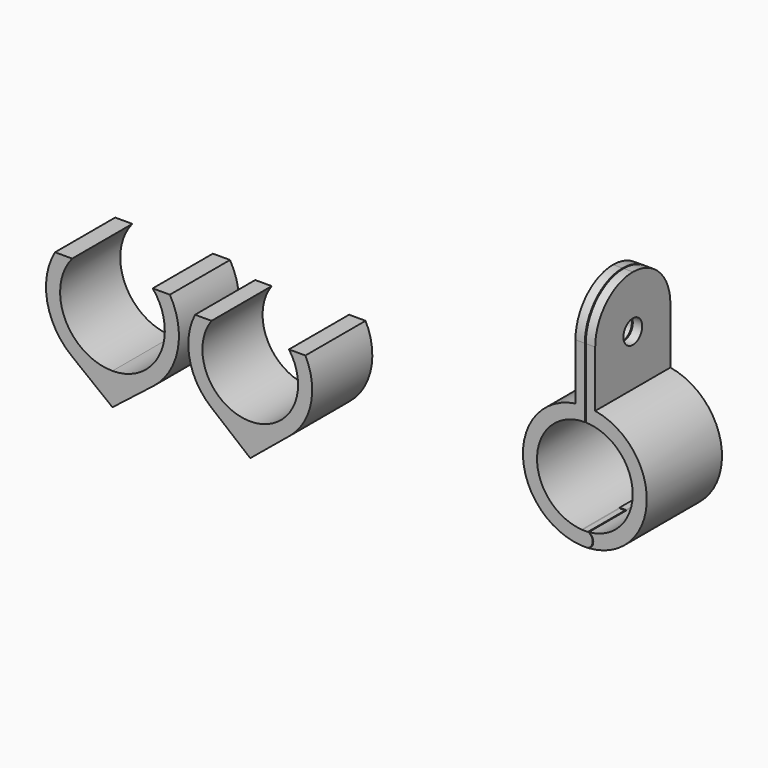
from build123d import *

# Parameters (mm, degrees)
F5_DEPTH  = 5
F0_R      = 0.45
F6_DEPTH  = 3.5
F7_DEPTH  = 5
F8_DEPTH  = 3.3
F9_DEPTH  = 5.001
F10_DEPTH = 8.001
F11_DEPTH = 0.05
F12_R     = 1.25
F13_DEPTH = 62.4297639076
F14_R     = 4.99999


# Not quite as in the source:
# - a fillet or chamfer is up to 0.001 mm smaller than in the source, because OpenCascade refuses the exact size
# - a feature names something its author has since deleted; it is built from what else it names


with BuildPart() as f3:
    # F3: sweep along a path in F2
    with BuildLine(Plane.XY) as f3_path:
        Line((0, 0), (0, 8))
    # F0 (on Front) → F3 (sweep)
    with BuildSketch(Plane.XZ):
        with BuildLine():
            Line((-4.2852259595, 12.5322833964), (-6.1092684933, 12.5322833964))
            ThreePointArc((-6.1092684933, 12.5322833964), (-6.9428544736, 7.6391569536), (-4.3543082114, 3.4039497307))
            Line((-4.3543082114, 3.4039497307), (0, 3.4039497307))
            ThreePointArc((0, 3.4039497307), (-5.042063988, 6.6069916109), (-4.2852259595, 12.5322833964))
        make_face()
        with BuildLine():
            Line((0, 3.4039497307), (-4.3543082114, 3.4039497307))
            ThreePointArc((-4.3543082114, 3.4039497307), (-2.3027157879, 2.2894602214), (0, 1.9039497307))
            Line((0, 1.9039497307), (0, 3.4039497307))
        make_face()
        with BuildLine():
            ThreePointArc((0, 1.9039497307), (-2.3027157879, 2.2894602214), (-4.3543082114, 3.4039497307))
            Line((-4.3543082114, 3.4039497307), (0, 0))
            Line((0, 0), (0, 1.9039497307))
        make_face()
        with BuildLine():
            ThreePointArc((4.3543082114, 3.4039497307), (2.3027157879, 2.2894602214), (0, 1.9039497307))
            Line((0, 1.9039497307), (0, 0))
            Line((0, 0), (4.3543082114, 3.4039497307))
        make_face()
        with BuildLine():
            Line((0, 3.4039497307), (0, 1.9039497307))
            ThreePointArc((0, 1.9039497307), (2.3027157879, 2.2894602214), (4.3543082114, 3.4039497307))
            Line((4.3543082114, 3.4039497307), (0, 3.4039497307))
        make_face()
        with BuildLine():
            ThreePointArc((4.2852259595, 12.5322833964), (5.042063988, 6.6069916109), (0, 3.4039497307))
            Line((0, 3.4039497307), (4.3543082114, 3.4039497307))
            ThreePointArc((4.3543082114, 3.4039497307), (6.9428544736, 7.6391569536), (6.1092684933, 12.5322833964))
            Line((6.1092684933, 12.5322833964), (4.2852259595, 12.5322833964))
        make_face()
    sweep(path=f3_path.line)

    # F0 (on Front) → F9 (cut, through all)
    with BuildSketch(Plane.XZ):
        with BuildLine():
            ThreePointArc((54.5868154242, 8.1161158316), (55.0876267464, 7.3630999101), (54.581783754, 6.6134547771))
            ThreePointArc((54.581783754, 6.6134547771), (54.6381547588, 6.6164632985), (54.6944979239, 6.6199545901))
            ThreePointArc((54.6944979239, 6.6199545901), (55.1524674782, 7.3759380646), (54.6800855939, 8.1230006335))
            ThreePointArc((54.6800855939, 8.1230006335), (54.6334663221, 8.1193440091), (54.5868154242, 8.1161158316))
        make_face()
    extrude(amount=F9_DEPTH, mode=Mode.SUBTRACT)

    # F0 (on Front) → F10 (cut, through all)
    with BuildSketch(Plane.XZ):
        with BuildLine():
            ThreePointArc((53.9199314878, 8.116823601), (53.3614179699, 7.3872965022), (53.862876759, 6.6174353327))
            ThreePointArc((53.862876759, 6.6174353327), (53.9147482987, 6.6145187306), (53.9666412198, 6.6120111547))
            ThreePointArc((53.9666412198, 6.6120111547), (53.4175421646, 7.3754821716), (54.0022997363, 8.1119985313))
            ThreePointArc((54.0022997363, 8.1119985313), (53.961105835, 8.1142441636), (53.9199314878, 8.116823601))
        make_face()
    extrude(amount=-F10_DEPTH, mode=Mode.SUBTRACT)


with BuildPart() as f4:
    # F4: sweep along a path in F2
    with BuildLine(Plane.XY) as f4_path:
        Line((14.6589075401, 0), (14.6589075401, 8))
    # F0 (on Front) → F4 (sweep)
    with BuildSketch(Plane.XZ):
        with BuildLine():
            Line((10.542163481, 11.5254557146), (8.7879977598, 11.5254557146))
            ThreePointArc((8.7879977598, 11.5254557146), (8.2076139721, 7.1870854906), (10.4732176329, 3.442043222))
            Line((10.4732176329, 3.442043222), (14.6589075401, 3.442043222))
            ThreePointArc((14.6589075401, 3.442043222), (10.1232394754, 6.2221048665), (10.542163481, 11.5254557146))
        make_face()
        with BuildLine():
            Line((14.6589075401, 3.442043222), (10.4732176329, 3.442043222))
            ThreePointArc((10.4732176329, 3.442043222), (12.4357341326, 2.3283668926), (14.6589075401, 1.942043222))
            Line((14.6589075401, 1.942043222), (14.6589075401, 3.442043222))
        make_face()
        with BuildLine():
            ThreePointArc((14.6589075401, 1.942043222), (12.4357341326, 2.3283668926), (10.4732176329, 3.442043222))
            Line((10.4732176329, 3.442043222), (14.6589075401, 0))
            Line((14.6589075401, 0), (14.6589075401, 1.942043222))
        make_face()
        with BuildLine():
            ThreePointArc((18.8445974474, 3.442043222), (16.8820809477, 2.3283668926), (14.6589075401, 1.942043222))
            Line((14.6589075401, 1.942043222), (14.6589075401, 0))
            Line((14.6589075401, 0), (18.8445974474, 3.442043222))
        make_face()
        with BuildLine():
            Line((14.6589075401, 3.442043222), (14.6589075401, 1.942043222))
            ThreePointArc((14.6589075401, 1.942043222), (16.8820809477, 2.3283668926), (18.8445974474, 3.442043222))
            Line((18.8445974474, 3.442043222), (14.6589075401, 3.442043222))
        make_face()
        with BuildLine():
            ThreePointArc((18.7756515993, 11.5254557146), (19.1945756049, 6.2221048665), (14.6589075401, 3.442043222))
            Line((14.6589075401, 3.442043222), (18.8445974474, 3.442043222))
            ThreePointArc((18.8445974474, 3.442043222), (21.1102011082, 7.1870854906), (20.5298173205, 11.5254557146))
            Line((20.5298173205, 11.5254557146), (18.7756515993, 11.5254557146))
        make_face()
    sweep(path=f4_path.line)


with BuildPart() as f5:
    # F0 (on Front) → F5 (new body)
    with BuildSketch(Plane.XZ):
        with BuildLine():
            Line((53.2587639076, 18.1863348766), (53.2587639076, 19.7092189305))
            ThreePointArc((53.2587639076, 19.7092189305), (47.6757687932, 12.8917648009), (53.862876759, 6.6174353327))
            ThreePointArc((53.862876759, 6.6174353327), (53.3614179699, 7.3872965022), (53.9199314878, 8.116823601))
            ThreePointArc((53.9199314878, 8.116823601), (49.1797007662, 12.8620403018), (53.2587639076, 18.1863348766))
        make_face()
        with BuildLine():
            Line((53.2587639076, 30.67503149), (53.2587639076, 19.7092189305))
            Line((53.2587639076, 19.7092189305), (53.2587639076, 18.1863348766))
            ThreePointArc((53.2587639076, 18.1863348766), (53.7563098464, 18.2606730117), (54.2587639076, 18.2855333378))
            Line((54.2587639076, 18.2855333378), (54.2587639076, 30.67503149))
            Line((54.2587639076, 30.67503149), (53.2587639076, 30.67503149))
        make_face()
    extrude(amount=-F5_DEPTH)



with BuildPart() as f5b:
    # F0 (on Front) → F5, piece 2 (new body)
    with BuildSketch(Plane.XZ):
        with BuildLine():
            ThreePointArc((54.0022997363, 8.1119985313), (53.4175421646, 7.3754821716), (53.9666412198, 6.6120111547))
            ThreePointArc((53.9666412198, 6.6120111547), (54.1126666567, 6.6071529911), (54.2587639076, 6.6055333378))
            Line((54.2587639076, 6.6055333378), (54.2587639076, 6.8555333378))
            ThreePointArc((54.2587639076, 6.8555333378), (53.7587639076, 7.3555333378), (54.2587639076, 7.8555333378))
            Line((54.2587639076, 7.8555333378), (54.2587639076, 8.1055333378))
            ThreePointArc((54.2587639076, 8.1055333378), (54.1304910833, 8.1071498929), (54.0022997363, 8.1119985313))
        make_face()
        with BuildLine():
            Line((54.2587639076, 6.8555333378), (54.2587639076, 6.6055333378))
            ThreePointArc((54.2587639076, 6.6055333378), (54.420322388, 6.6075139953), (54.581783754, 6.6134547771))
            ThreePointArc((54.581783754, 6.6134547771), (55.0876267464, 7.3630999101), (54.5868154242, 8.1161158316))
            ThreePointArc((54.5868154242, 8.1161158316), (54.4228749879, 8.1081796492), (54.2587639076, 8.1055333378))
            Line((54.2587639076, 8.1055333378), (54.2587639076, 7.8555333378))
            ThreePointArc((54.2587639076, 7.8555333378), (54.6123172982, 7.7090867284), (54.7587639076, 7.3555333378))
            ThreePointArc((54.7587639076, 7.3555333378), (54.6123172982, 7.0019799472), (54.2587639076, 6.8555333378))
        make_face()
        with BuildLine():
            ThreePointArc((54.5868154242, 8.1161158316), (55.0876267464, 7.3630999101), (54.581783754, 6.6134547771))
            ThreePointArc((54.581783754, 6.6134547771), (54.6381547588, 6.6164632985), (54.6944979239, 6.6199545901))
            ThreePointArc((54.6944979239, 6.6199545901), (55.1524674782, 7.3759380646), (54.6800855939, 8.1230006335))
            ThreePointArc((54.6800855939, 8.1230006335), (54.6334663221, 8.1193440091), (54.5868154242, 8.1161158316))
        make_face()
        with BuildLine():
            ThreePointArc((54.2587639076, 7.8555333378), (53.7587639076, 7.3555333378), (54.2587639076, 6.8555333378))
            ThreePointArc((54.2587639076, 6.8555333378), (54.6123172982, 7.0019799472), (54.7587639076, 7.3555333378))
            ThreePointArc((54.7587639076, 7.3555333378), (54.6123172982, 7.7090867284), (54.2587639076, 7.8555333378))
        make_face()
        with Locations((54.2587639076, 7.3555333378)):
            Circle(F0_R, mode=Mode.SUBTRACT)
        with BuildLine():
            ThreePointArc((54.6800855939, 8.1230006335), (55.1524674782, 7.3759380646), (54.6944979239, 6.6199545901))
            ThreePointArc((54.6944979239, 6.6199545901), (60.8402732623, 12.8611165114), (55.3587639076, 19.6930790283))
            Line((55.3587639076, 19.6930790283), (55.3587639076, 18.1652516397))
            ThreePointArc((55.3587639076, 18.1652516397), (59.3371796287, 12.8523223769), (54.6800855939, 8.1230006335))
        make_face()
        with BuildLine():
            Line((55.3587639076, 18.1652516397), (55.3587639076, 19.6930790283))
            Line((55.3587639076, 19.6930790283), (55.3587639076, 30.67503149))
            Line((55.3587639076, 30.67503149), (54.3587639076, 30.67503149))
            Line((54.3587639076, 30.67503149), (54.3587639076, 18.2845509247))
            ThreePointArc((54.3587639076, 18.2845509247), (54.8617216838, 18.24969419), (55.3587639076, 18.1652516397))
        make_face()
        with Locations((54.2587639076, 7.3555333378)):
            Circle(F0_R)
    extrude(amount=-F5_DEPTH)

    # F0 (on Front) → F6 (cut)
    with BuildSketch(Plane.XZ):
        with BuildLine():
            ThreePointArc((54.2587639076, 7.8555333378), (53.7587639076, 7.3555333378), (54.2587639076, 6.8555333378))
            ThreePointArc((54.2587639076, 6.8555333378), (54.6123172982, 7.0019799472), (54.7587639076, 7.3555333378))
            ThreePointArc((54.7587639076, 7.3555333378), (54.6123172982, 7.7090867284), (54.2587639076, 7.8555333378))
        make_face()
        with Locations((54.2587639076, 7.3555333378)):
            Circle(F0_R, mode=Mode.SUBTRACT)
        with Locations((54.2587639076, 7.3555333378)):
            Circle(F0_R)
    extrude(amount=-F6_DEPTH, mode=Mode.SUBTRACT)


with BuildPart() as f5_1:
    add(f5.part)

    add(f5b.part)  # F7 merges F5b
    # F0 (on Front) → F7 (join)
    with BuildSketch(Plane.XZ):
        with BuildLine():
            Line((53.2587639076, 18.1863348766), (53.2587639076, 19.7092189305))
            ThreePointArc((53.2587639076, 19.7092189305), (47.6757687932, 12.8917648009), (53.862876759, 6.6174353327))
            ThreePointArc((53.862876759, 6.6174353327), (53.3614179699, 7.3872965022), (53.9199314878, 8.116823601))
            ThreePointArc((53.9199314878, 8.116823601), (49.1797007662, 12.8620403018), (53.2587639076, 18.1863348766))
        make_face()
        with BuildLine():
            Line((53.2587639076, 30.67503149), (53.2587639076, 19.7092189305))
            Line((53.2587639076, 19.7092189305), (53.2587639076, 18.1863348766))
            ThreePointArc((53.2587639076, 18.1863348766), (53.7563098464, 18.2606730117), (54.2587639076, 18.2855333378))
            Line((54.2587639076, 18.2855333378), (54.2587639076, 30.67503149))
            Line((54.2587639076, 30.67503149), (53.2587639076, 30.67503149))
        make_face()
        with BuildLine():
            ThreePointArc((53.9199314878, 8.116823601), (53.3614179699, 7.3872965022), (53.862876759, 6.6174353327))
            ThreePointArc((53.862876759, 6.6174353327), (53.9147482987, 6.6145187306), (53.9666412198, 6.6120111547))
            ThreePointArc((53.9666412198, 6.6120111547), (53.4175421646, 7.3754821716), (54.0022997363, 8.1119985313))
            ThreePointArc((54.0022997363, 8.1119985313), (53.961105835, 8.1142441636), (53.9199314878, 8.116823601))
        make_face()
        with BuildLine():
            ThreePointArc((54.0022997363, 8.1119985313), (53.4175421646, 7.3754821716), (53.9666412198, 6.6120111547))
            ThreePointArc((53.9666412198, 6.6120111547), (54.1126666567, 6.6071529911), (54.2587639076, 6.6055333378))
            Line((54.2587639076, 6.6055333378), (54.2587639076, 6.8555333378))
            ThreePointArc((54.2587639076, 6.8555333378), (53.7587639076, 7.3555333378), (54.2587639076, 7.8555333378))
            Line((54.2587639076, 7.8555333378), (54.2587639076, 8.1055333378))
            ThreePointArc((54.2587639076, 8.1055333378), (54.1304910833, 8.1071498929), (54.0022997363, 8.1119985313))
        make_face()
        with BuildLine():
            Line((54.2587639076, 6.8555333378), (54.2587639076, 6.6055333378))
            ThreePointArc((54.2587639076, 6.6055333378), (54.420322388, 6.6075139953), (54.581783754, 6.6134547771))
            ThreePointArc((54.581783754, 6.6134547771), (55.0876267464, 7.3630999101), (54.5868154242, 8.1161158316))
            ThreePointArc((54.5868154242, 8.1161158316), (54.4228749879, 8.1081796492), (54.2587639076, 8.1055333378))
            Line((54.2587639076, 8.1055333378), (54.2587639076, 7.8555333378))
            ThreePointArc((54.2587639076, 7.8555333378), (54.6123172982, 7.7090867284), (54.7587639076, 7.3555333378))
            ThreePointArc((54.7587639076, 7.3555333378), (54.6123172982, 7.0019799472), (54.2587639076, 6.8555333378))
        make_face()
        with BuildLine():
            ThreePointArc((54.2587639076, 7.8555333378), (53.7587639076, 7.3555333378), (54.2587639076, 6.8555333378))
            ThreePointArc((54.2587639076, 6.8555333378), (54.6123172982, 7.0019799472), (54.7587639076, 7.3555333378))
            ThreePointArc((54.7587639076, 7.3555333378), (54.6123172982, 7.7090867284), (54.2587639076, 7.8555333378))
        make_face()
        with Locations((54.2587639076, 7.3555333378)):
            Circle(F0_R, mode=Mode.SUBTRACT)
        with BuildLine():
            ThreePointArc((54.6800855939, 8.1230006335), (55.1524674782, 7.3759380646), (54.6944979239, 6.6199545901))
            ThreePointArc((54.6944979239, 6.6199545901), (60.8402732623, 12.8611165114), (55.3587639076, 19.6930790283))
            Line((55.3587639076, 19.6930790283), (55.3587639076, 18.1652516397))
            ThreePointArc((55.3587639076, 18.1652516397), (59.3371796287, 12.8523223769), (54.6800855939, 8.1230006335))
        make_face()
        with BuildLine():
            Line((55.3587639076, 18.1652516397), (55.3587639076, 19.6930790283))
            Line((55.3587639076, 19.6930790283), (55.3587639076, 30.67503149))
            Line((55.3587639076, 30.67503149), (54.3587639076, 30.67503149))
            Line((54.3587639076, 30.67503149), (54.3587639076, 18.2845509247))
            ThreePointArc((54.3587639076, 18.2845509247), (54.8617216838, 18.24969419), (55.3587639076, 18.1652516397))
        make_face()
        with Locations((54.2587639076, 7.3555333378)):
            Circle(F0_R)
    extrude(amount=F7_DEPTH)

    # F0 (on Front) → F8 (join)
    with BuildSketch(Plane.XZ):
        with Locations((54.2587639076, 7.3555333378)):
            Circle(F0_R)
    extrude(amount=-F8_DEPTH)

    # F0 (on Front) → F11 (cut, symmetric)
    with BuildSketch(Plane.XZ):
        with BuildLine():
            Line((54.2587639076, 6.8555333378), (54.2587639076, 6.6055333378))
            ThreePointArc((54.2587639076, 6.6055333378), (54.420322388, 6.6075139953), (54.581783754, 6.6134547771))
            ThreePointArc((54.581783754, 6.6134547771), (55.0876267464, 7.3630999101), (54.5868154242, 8.1161158316))
            ThreePointArc((54.5868154242, 8.1161158316), (54.4228749879, 8.1081796492), (54.2587639076, 8.1055333378))
            Line((54.2587639076, 8.1055333378), (54.2587639076, 7.8555333378))
            ThreePointArc((54.2587639076, 7.8555333378), (54.6123172982, 7.7090867284), (54.7587639076, 7.3555333378))
            ThreePointArc((54.7587639076, 7.3555333378), (54.6123172982, 7.0019799472), (54.2587639076, 6.8555333378))
        make_face()
        with BuildLine():
            ThreePointArc((54.0022997363, 8.1119985313), (53.4175421646, 7.3754821716), (53.9666412198, 6.6120111547))
            ThreePointArc((53.9666412198, 6.6120111547), (54.1126666567, 6.6071529911), (54.2587639076, 6.6055333378))
            Line((54.2587639076, 6.6055333378), (54.2587639076, 6.8555333378))
            ThreePointArc((54.2587639076, 6.8555333378), (53.7587639076, 7.3555333378), (54.2587639076, 7.8555333378))
            Line((54.2587639076, 7.8555333378), (54.2587639076, 8.1055333378))
            ThreePointArc((54.2587639076, 8.1055333378), (54.1304910833, 8.1071498929), (54.0022997363, 8.1119985313))
        make_face()
    extrude(amount=F11_DEPTH, both=True, mode=Mode.SUBTRACT)

    # F12 (on face) → F13 (cut, through all)
    with BuildSketch(Plane.YZ.offset(55.3587639076)):
        with Locations((0, 25.0911675394)):
            Circle(F12_R)
    extrude(amount=-F13_DEPTH, mode=Mode.SUBTRACT)

    # F14 (radius 5 in the source; OpenCascade refuses exactly that, so slightly less here)
    f14_edges = [f5_1.edges().sort_by_distance(p)[0] for p in [
        (53.758764, -5, 30.675031),
        (54.858764, -5, 30.675031),
        (53.758764, 5, 30.675031),
        (54.858764, 5, 30.675031),
    ]]
    fillet(f14_edges, radius=F14_R)


solid = Compound([f3.part, f4.part, f5_1.part])
